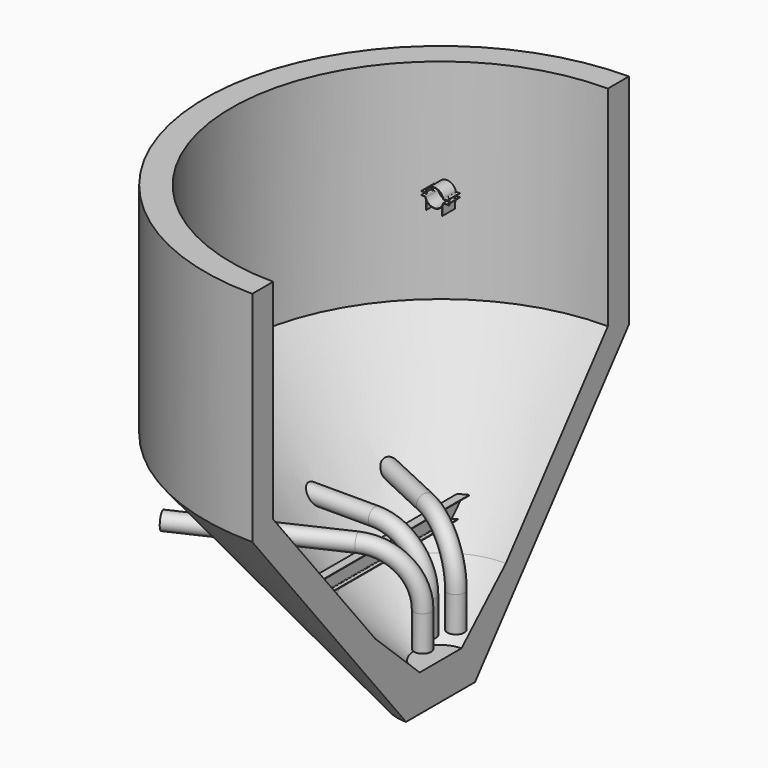
from build123d import *

# Parameters (mm, degrees)
F1_DEPTH       = 150
F1_DEPTH_BACK  = 150
F3_ANGLE_BACK  = 90
F3_ANGLE       = 180
F4_DEPTH       = 2000
F4_DEPTH_BACK  = 2000
F13_R          = 10
F14_DEPTH      = 120
F14_DEPTH_BACK = 1
F11_R          = 161.95
F11_R_2        = 141.95
F12_R          = 161.95
F12_R_2        = 141.95
F10_R          = 161.95
F10_R_2        = 141.95


# Not quite as in the source:
# - a feature of the source that left no trace in its solid (it failed there, or was rolled back) is left out
# - a pattern or mirror of a feature is missing from the dataset's text; its kind, count and spacing are read off the source's solid


with BuildPart() as f1:
    # F0 (on Front) → F1 (new body, two sides)
    with BuildSketch(Plane.XZ) as f1_sk:
        with BuildLine():
            Line((-247.3320053068, 38), (-247.3320053068, 30))
            Line((-247.3320053068, 30), (-179.4435844493, 30))
            ThreePointArc((-179.4435844493, 30), (-170.2167141708, 33.1735523142), (-164.8941046291, 41.3513513514))
            ThreePointArc((-164.8941046291, 41.3513513514), (-104.571196489, 134.0330737724), (0, 170))
            ThreePointArc((0, 170), (104.571196489, 134.0330737724), (164.8941046291, 41.3513513514))
            ThreePointArc((164.8941046291, 41.3513513514), (170.2167141708, 33.1735523142), (179.4435844493, 30))
            Line((179.4435844493, 30), (247.3320053068, 30))
            Line((247.3320053068, 30), (247.3320053068, 38))
            Line((247.3320053068, 38), (185.5801713546, 38))
            ThreePointArc((185.5801713546, 38), (176.5465553778, 41.0252857076), (171.1568419747, 48.8808290155))
            ThreePointArc((171.1568419747, 48.8808290155), (165.4082002886, 65.7580966671), (158, 81.9756061277))
            ThreePointArc((158, 81.9756061277), (92.4455031607, 152.1112387214), (0, 178))
            ThreePointArc((0, 178), (-92.4455031607, 152.1112387214), (-158, 81.9756061277))
            ThreePointArc((-158, 81.9756061277), (-165.4082002886, 65.7580966671), (-171.1568419747, 48.8808290155))
            ThreePointArc((-171.1568419747, 48.8808290155), (-176.5465553778, 41.0252857076), (-185.5801713546, 38))
            Line((-185.5801713546, 38), (-247.3320053068, 38))
        make_face()
    extrude(amount=F1_DEPTH)
    extrude(f1_sk.sketch, amount=-F1_DEPTH_BACK)



with BuildPart() as f1b:
    # F0 (on Front) → F1, piece 2 (new body, two sides)
    with BuildSketch(Plane.XZ) as f1_2_sk:
        with BuildLine():
            ThreePointArc((179.4435844493, -30), (170.2167141708, -33.1735523142), (164.8941046291, -41.3513513514))
            ThreePointArc((164.8941046291, -41.3513513514), (104.571196489, -134.0330737724), (0, -170))
            ThreePointArc((0, -170), (-104.571196489, -134.0330737724), (-164.8941046291, -41.3513513514))
            ThreePointArc((-164.8941046291, -41.3513513514), (-170.2167141708, -33.1735523142), (-179.4435844493, -30))
            Line((-179.4435844493, -30), (-247.3320053068, -30))
            Line((-247.3320053068, -30), (-247.3320053068, -38))
            Line((-247.3320053068, -38), (-185.5801713546, -38))
            ThreePointArc((-185.5801713546, -38), (-176.5465553778, -41.0252857076), (-171.1568419747, -48.8808290155))
            ThreePointArc((-171.1568419747, -48.8808290155), (-165.4082002886, -65.7580966671), (-158, -81.9756061277))
            Line((-158, -81.9756061277), (-158, -251.9756061277))
            Line((-158, -251.9756061277), (-150, -251.9756061277))
            Line((-150, -251.9756061277), (-150, -95.8331884057))
            ThreePointArc((-150, -95.8331884057), (-85.5151812949, -156.1126316738), (0, -178))
            ThreePointArc((0, -178), (85.5151812949, -156.1126316738), (150, -95.8331884057))
            Line((150, -95.8331884057), (150, -251.9756061277))
            Line((150, -251.9756061277), (158, -251.9756061277))
            Line((158, -251.9756061277), (158, -81.9756061277))
            ThreePointArc((158, -81.9756061277), (165.4082002886, -65.7580966671), (171.1568419747, -48.8808290155))
            ThreePointArc((171.1568419747, -48.8808290155), (176.5465553778, -41.0252857076), (185.5801713546, -38))
            Line((185.5801713546, -38), (247.3320053068, -38))
            Line((247.3320053068, -38), (247.3320053068, -30))
            Line((247.3320053068, -30), (179.4435844493, -30))
        make_face()
    extrude(amount=F1_DEPTH)
    extrude(f1_2_sk.sketch, amount=-F1_DEPTH_BACK)


with BuildPart() as f3:
    # F2 (on Front) → F3 (revolve)
    with BuildSketch(Plane.XZ, mode=Mode.PRIVATE) as f3_sk:
        Polygon((-4000, 153.5), (-4500, 153.5), (-4500, -4024.0485725608), (-824.7544733011, -8546.5), (0, -8546.5), (0, -7846.5), (-500, -7846.5), (-1562, -6846.5), (-4000, -3846.5), align=None)
    revolve(f3_sk.sketch.rotate(Axis((0, 0, -4846.3342590332), (0, 0, -1)), -F3_ANGLE_BACK), axis=Axis((0, 0, -4846.3342590332), (0, 0, -1)), revolution_arc=F3_ANGLE)

    # F2 (on Front) → F4 (join, two sides)
    with BuildSketch(Plane.XZ) as f4_sk:
        with BuildLine():
            Line((-967.5, -6146.5), (-1132.5, -6146.5))
            Line((-1132.5, -6146.5), (-1132.5, -6156.7))
            Line((-1132.5, -6156.7), (-1064.45, -6156.7))
            ThreePointArc((-1064.45, -6156.7), (-1056.3889826945, -6160.0389826945), (-1053.05, -6168.1))
            Line((-1053.05, -6168.1), (-1053.05, -6431.9))
            ThreePointArc((-1053.05, -6431.9), (-1056.3889826945, -6439.9610173055), (-1064.45, -6443.3))
            Line((-1064.45, -6443.3), (-1132.5, -6443.3))
            Line((-1132.5, -6443.3), (-1132.5, -6453.5))
            Line((-1132.5, -6453.5), (-967.5, -6453.5))
            Line((-967.5, -6453.5), (-967.5, -6443.3))
            Line((-967.5, -6443.3), (-1035.55, -6443.3))
            ThreePointArc((-1035.55, -6443.3), (-1043.6110173055, -6439.9610173055), (-1046.95, -6431.9))
            Line((-1046.95, -6431.9), (-1046.95, -6168.1))
            ThreePointArc((-1046.95, -6168.1), (-1043.6110173055, -6160.0389826945), (-1035.55, -6156.7))
            Line((-1035.55, -6156.7), (-967.5, -6156.7))
            Line((-967.5, -6156.7), (-967.5, -6146.5))
        make_face()
    extrude(amount=F4_DEPTH)
    extrude(f4_sk.sketch, amount=-F4_DEPTH_BACK)

    # F20: sweep along a path in F19
    with BuildLine(Plane.XZ) as f20_path:
        Line((-3650, -5826.5), (-1250, -5826.5))
        ThreePointArc((-1250, -5826.5), (-542.8932188135, -6119.3932188135), (-250, -6826.5))
        Line((-250, -6826.5), (-250, -7496.5))
    # F11 (on line) → F20 (sweep)
    with BuildSketch(Plane(origin=(-3650, 0, 0), x_dir=(0, -1, 0), z_dir=(-1, 0, 0))):
        with Locations((0, -5826.5)):
            Circle(F11_R)
        with Locations((0, -5826.5)):
            Circle(F11_R_2, mode=Mode.SUBTRACT)
    sweep(path=f20_path.line)

    # F22: sweep along a path in F21
    with BuildLine(Plane(origin=(147.9163916092, -317.2077254628, 0), x_dir=(-0.906307787, -0.4226182617, 0), z_dir=(-0.4226182617, 0.906307787, 0))) as f22_path:
        Line((4190.5370845674, -5826.5), (1190.5370845673, -5826.5))
        ThreePointArc((1190.5370845673, -5826.5), (483.4303033808, -6119.3932188135), (190.5370845673, -6826.5))
        Line((190.5370845673, -6826.5), (190.5370845673, -7496.5))
    # F12 (on line) → F22 (sweep)
    with BuildSketch(Plane(origin=(-3797.9163916092, -1770.9974984398, 0), x_dir=(-0.4226182617, 0.906307787, 0), z_dir=(0.906307787, 0.4226182617, 0))):
        with Locations((-350, -5826.5)):
            Circle(F12_R)
        with Locations((-350, -5826.5)):
            Circle(F12_R_2, mode=Mode.SUBTRACT)
    sweep(path=f22_path.line)

    # F24: sweep along a path in F23
    with BuildLine(Plane(origin=(147.9163916092, 317.2077254628, 0), x_dir=(-0.906307787, 0.4226182617, 0), z_dir=(0.4226182617, 0.906307787, 0))) as f24_path:
        Line((4190.5370845674, -5826.5), (1190.5370845673, -5826.5))
        ThreePointArc((1190.5370845673, -5826.5), (483.4303033808, -6119.3932188135), (190.5370845673, -6826.5))
        Line((190.5370845673, -6826.5), (190.5370845673, -7496.5))
    # F10 (on line) → F24 (sweep)
    with BuildSketch(Plane(origin=(-3797.9163916092, 1770.9974984398, 0), x_dir=(0.4226182617, 0.906307787, 0), z_dir=(0.906307787, -0.4226182617, 0))):
        with Locations((350, -5826.5)):
            Circle(F10_R)
        with Locations((350, -5826.5)):
            Circle(F10_R_2, mode=Mode.SUBTRACT)
    sweep(path=f24_path.line)


with BuildPart() as f1_1:
    add(f1.part)

    add(f1b.part)  # F14 merges F1b
    # F13 (on face) → F14 (join, two sides)
    with BuildSketch(Plane.XY.offset(38)) as f14_sk:
        with Locations((-216.4560883307, 75)):
            Circle(F13_R)
    f14 = extrude(amount=-F14_DEPTH) + extrude(f14_sk.sketch, amount=F14_DEPTH_BACK)

    # F14_copies: F14 across plane
    add(f14.mirror(Plane(origin=(0, 0, 0), x_dir=(0, 0, -1), z_dir=(0, -1, 0))))

    # F14_copies1: F14 across plane
    add(f14.mirror(Plane(origin=(0, 0, 0), x_dir=(0, 0, 1), z_dir=(1, 0, 0))))

    # F14_copies2: F14 across plane
    add(f14.mirror(Plane(origin=(0, 0, 0), x_dir=(0.3273946967, 0.9448876719, 0), z_dir=(0.9448876719, -0.3273946967, 0))))


solid = Compound([f3.part, f1_1.part])
